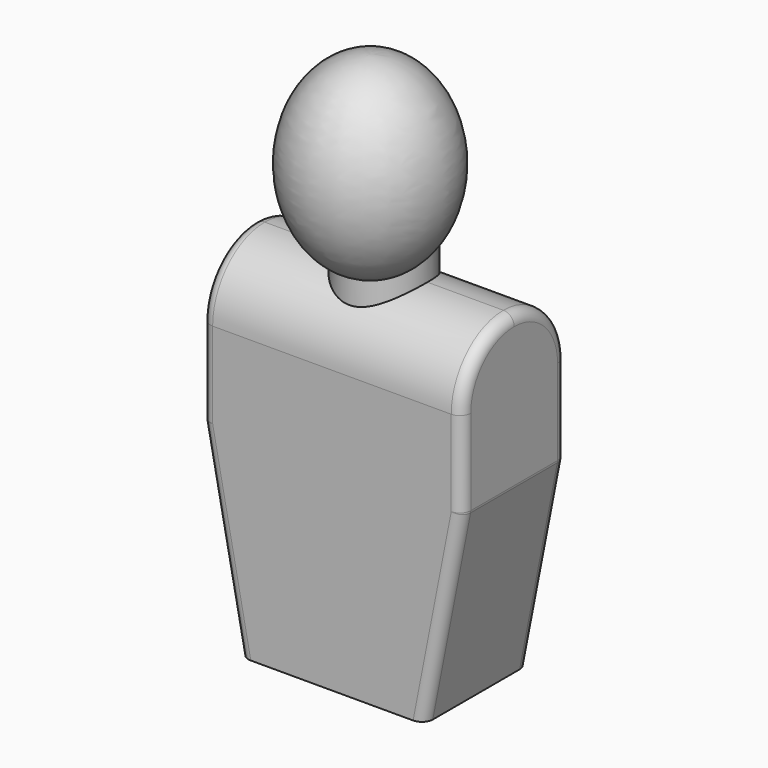
from build123d import *

# Parameters (mm, degrees)
F1_DEPTH    = 19.05
F2_T1_DEPTH = 171.45
F3_W        = 12.7
F3_H        = 38.1
F7_R        = 3.175
F8_R        = 3.175


# Not quite as in the source:
# - a fillet or chamfer that OpenCascade refuses, or shapes differently, is made with other operations: its cross-section is extruded or revolved along the edge and cut away or added


with BuildPart() as f1:
    # F0 (on Front) → F1 (new body, symmetric)
    with BuildSketch(Plane.XZ):
        Polygon((-38.1, 57.15), (-26.9875, 0), (26.9875, 0), (38.1, 57.15), (38.1, 101.6), (-38.1, 101.6), align=None)
    extrude(amount=F1_DEPTH, both=True)

    # F2: fillet of radius 19.05 on 2 edges, made by hand

    # F2_s2 → F2_t1 (cut)
    with BuildSketch(Plane.YZ.offset(-85.725)):
        with BuildLine():
            ThreePointArc((0, 101.6), (-13.4703841816, 96.0203841816), (-19.05, 82.55))
            Line((-19.05, 82.55), (-19.05, 101.6))
            Line((-19.05, 101.6), (0, 101.6))
        make_face()
        with BuildLine():
            ThreePointArc((0, 101.6), (13.4703841816, 96.0203841816), (19.05, 82.55))
            Line((19.05, 82.55), (19.05, 101.6))
            Line((19.05, 101.6), (0, 101.6))
        make_face()
    extrude(amount=F2_T1_DEPTH, mode=Mode.SUBTRACT)

    # F3 (on Front) → F4 (revolve)
    with BuildSketch(Plane.XZ):
        with Locations((6.35, 101.6)):
            Rectangle(F3_W, F3_H)
    revolve(axis=Axis((0, 0, 41.275), (0, 0, -1)))

    # F5 (on Right) → F6 (revolve)
    with BuildSketch(Plane.YZ):
        with BuildLine():
            Line((-5.08, 158.115), (-5.08, 102.235))
            add(Edge.make_bspline(
                [(-5.08, 102.235), (17.145, 102.235), (17.145, 130.175), (17.145, 158.115), (-5.08, 158.115)],
                knots=[3.1415926536, 3.1415926536, 3.1415926536, 4.7123889804, 4.7123889804, 6.2831853072, 6.2831853072, 6.2831853072], degree=2, weights=[1, 0.7071067812, 1, 0.7071067812, 1]))
        make_face()
    revolve(axis=Axis((0, -5.08, 55.275326029), (0, 0, -1)))

    # F7
    f7_edges = [f1.edges().sort_by_distance(p)[0] for p in [
        (-38.1, 0, 57.15),
        (38.1, 0, 57.15),
    ]]
    fillet(f7_edges, radius=F7_R)

    # F8
    f8_edges = [f1.edges().sort_by_distance(p)[0] for p in [
        (32.514564, -19.05, 28.424903),
        (-32.514564, -19.05, 28.424903),
        (-32.514564, 19.05, 28.424903),
        (-38.1, 19.05, 70.002908),
        (-38.085374, 19.05, 57.151409),
        (38.1, 19.05, 70.002908),
        (38.085374, 19.05, 57.151409),
        (32.514564, 19.05, 28.424903),
        (-38.085374, -19.05, 57.151409),
        (-38.1, -19.05, 70.002908),
        (38.1, -19.05, 70.002908),
        (38.085374, -19.05, 57.151409),
        (-38.1, -13.470384, 96.020384),
        (-38.1, 13.470384, 96.020384),
        (38.1, 13.470384, 96.020384),
        (38.1, -13.470384, 96.020384),
    ]]
    fillet(f8_edges, radius=F8_R)


solid = f1.part
